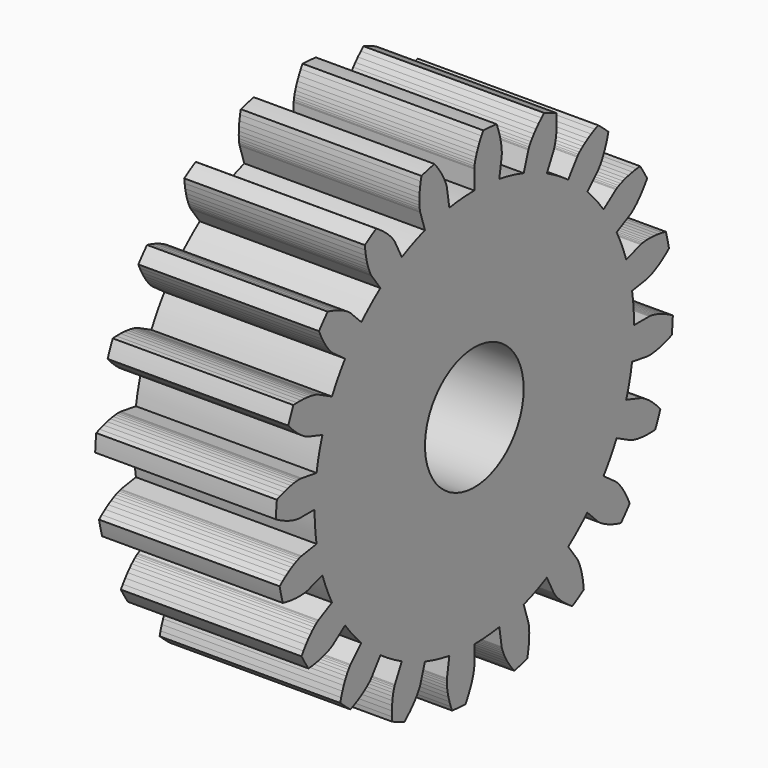
from build123d import *

# Parameters (mm, degrees)
F2_DEPTH = 12.7
F3_R     = 4.3353381976
F4_DEPTH = 12.701


# Not quite as in the source:
# - a variable given as a bare number and used for a length is read in inches; the dataset says mm whatever the document's units were


with BuildPart() as f2:
    # F1 (on Right) → F2 (new body)
    with BuildSketch(Plane.YZ):
        with BuildLine():
            ThreePointArc((13.8654281935, -2.1960680843), (13.9949872217, -1.1014293813), (14.0382625, 0))
            ThreePointArc((14.0382625, 0), (13.9949872217, 1.1014293813), (13.8654281935, 2.1960680843))
            ThreePointArc((13.8654281935, 2.1960680843), (13.6503841896, 3.2771672972), (13.3511810281, 4.338061684))
            ThreePointArc((13.3511810281, 4.338061684), (12.9696633958, 5.3722104779), (12.5081834758, 6.3732378078))
            ThreePointArc((12.5081834758, 6.3732378078), (11.9695864452, 7.3349720074), (11.357192934, 8.2514836653))
            ThreePointArc((11.357192934, 8.2514836653), (10.6747785517, 9.1171221826), (9.9265506098, 9.9265506098))
            ThreePointArc((9.9265506098, 9.9265506098), (9.1171221826, 10.6747785517), (8.2514836653, 11.357192934))
            ThreePointArc((8.2514836653, 11.357192934), (7.3349720074, 11.9695864452), (6.3732378078, 12.5081834758))
            ThreePointArc((6.3732378078, 12.5081834758), (5.3722104779, 12.9696633958), (4.338061684, 13.3511810281))
            ThreePointArc((4.338061684, 13.3511810281), (3.2771672972, 13.6503841896), (2.1960680843, 13.8654281935))
            ThreePointArc((2.1960680843, 13.8654281935), (1.1014293813, 13.9949872217), (0, 14.0382625))
            ThreePointArc((0, 14.0382625), (-1.1014293813, 13.9949872217), (-2.1960680843, 13.8654281935))
            ThreePointArc((-2.1960680843, 13.8654281935), (-3.2771672972, 13.6503841896), (-4.338061684, 13.3511810281))
            ThreePointArc((-4.338061684, 13.3511810281), (-5.3722104779, 12.9696633958), (-6.3732378078, 12.5081834758))
            ThreePointArc((-6.3732378078, 12.5081834758), (-7.3349720074, 11.9695864452), (-8.2514836653, 11.357192934))
            ThreePointArc((-8.2514836653, 11.357192934), (-9.1171221826, 10.6747785517), (-9.9265506098, 9.9265506098))
            ThreePointArc((-9.9265506098, 9.9265506098), (-10.6747785517, 9.1171221826), (-11.357192934, 8.2514836653))
            ThreePointArc((-11.357192934, 8.2514836653), (-11.9695864452, 7.3349720074), (-12.5081834758, 6.3732378078))
            ThreePointArc((-12.5081834758, 6.3732378078), (-12.9696633958, 5.3722104779), (-13.3511810281, 4.338061684))
            ThreePointArc((-13.3511810281, 4.338061684), (-13.6503841896, 3.2771672972), (-13.8654281935, 2.1960680843))
            ThreePointArc((-13.8654281935, 2.1960680843), (-13.9949872217, 1.1014293813), (-14.0382625, 0))
            ThreePointArc((-14.0382625, 0), (-13.9949872217, -1.1014293813), (-13.8654281935, -2.1960680843))
            ThreePointArc((-13.8654281935, -2.1960680843), (-13.6503841896, -3.2771672972), (-13.3511810281, -4.338061684))
            ThreePointArc((-13.3511810281, -4.338061684), (-12.9696633958, -5.3722104779), (-12.5081834758, -6.3732378078))
            ThreePointArc((-12.5081834758, -6.3732378078), (-11.9695864452, -7.3349720074), (-11.357192934, -8.2514836653))
            ThreePointArc((-11.357192934, -8.2514836653), (-10.6747785517, -9.1171221826), (-9.9265506098, -9.9265506098))
            ThreePointArc((-9.9265506098, -9.9265506098), (-9.1171221826, -10.6747785517), (-8.2514836653, -11.357192934))
            ThreePointArc((-8.2514836653, -11.357192934), (-7.3349720074, -11.9695864452), (-6.3732378078, -12.5081834758))
            ThreePointArc((-6.3732378078, -12.5081834758), (-5.3722104779, -12.9696633958), (-4.338061684, -13.3511810281))
            ThreePointArc((-4.338061684, -13.3511810281), (-3.2771672972, -13.6503841896), (-2.1960680843, -13.8654281935))
            ThreePointArc((-2.1960680843, -13.8654281935), (-1.1014293813, -13.9949872217), (0, -14.0382625))
            ThreePointArc((0, -14.0382625), (1.1014293813, -13.9949872217), (2.1960680843, -13.8654281935))
            ThreePointArc((2.1960680843, -13.8654281935), (3.2771672972, -13.6503841896), (4.338061684, -13.3511810281))
            ThreePointArc((4.338061684, -13.3511810281), (5.3722104779, -12.9696633958), (6.3732378078, -12.5081834758))
            ThreePointArc((6.3732378078, -12.5081834758), (7.3349720074, -11.9695864452), (8.2514836653, -11.357192934))
            ThreePointArc((8.2514836653, -11.357192934), (9.1171221826, -10.6747785517), (9.9265506098, -9.9265506098))
            ThreePointArc((9.9265506098, -9.9265506098), (10.6747785517, -9.1171221826), (11.357192934, -8.2514836653))
            ThreePointArc((11.357192934, -8.2514836653), (11.9695864452, -7.3349720074), (12.5081834758, -6.3732378078))
            ThreePointArc((12.5081834758, -6.3732378078), (12.9696633958, -5.3722104779), (13.3511810281, -4.338061684))
            ThreePointArc((13.3511810281, -4.338061684), (13.6503841896, -3.2771672972), (13.8654281935, -2.1960680843))
        make_face()
        with BuildLine():
            Line((-14.6171145636, -4.7493884238), (-13.3511810281, -4.338061684))
            ThreePointArc((-13.3511810281, -4.338061684), (-13.6503841896, -3.2771672972), (-13.8654281935, -2.1960680843))
            Line((-13.8654281935, -2.1960680843), (-15.180121665, -2.404295074))
            Line((-15.180121665, -2.404295074), (-15.1989848071, -2.4079309004))
            Line((-15.1989848071, -2.4079309004), (-15.2550320002, -2.4213414721))
            Line((-15.2550320002, -2.4213414721), (-15.3472398712, -2.4482306459))
            Line((-15.3472398712, -2.4482306459), (-15.474308977, -2.4922197725))
            Line((-15.474308977, -2.4922197725), (-15.6346697243, -2.5568294258))
            Line((-15.6346697243, -2.5568294258), (-15.8264894224, -2.6454615286))
            Line((-15.8264894224, -2.6454615286), (-16.0476804424, -2.7613819428))
            Line((-16.0476804424, -2.7613819428), (-16.2959094551, -2.9077035901))
            Line((-16.2959094551, -2.9077035901), (-16.5686077133, -3.0873701663))
            Line((-16.5686077133, -3.0873701663), (-16.8629823421, -3.3031405114))
            Line((-16.8629823421, -3.3031405114), (-17.1077308908, -3.5020636798))
            ThreePointArc((-17.1077308908, -3.5020636798), (-16.9800097349, -4.0765396663), (-16.8330034779, -4.6463857097))
            Line((-16.8330034779, -4.6463857097), (-16.5246216956, -4.7125140346))
            Line((-16.5246216956, -4.7125140346), (-16.1643742939, -4.771123535))
            Line((-16.1643742939, -4.771123535), (-15.8398314481, -4.807405208))
            Line((-15.8398314481, -4.807405208), (-15.5522291405, -4.8250851369))
            Line((-15.5522291405, -4.8250851369), (-15.3025197318, -4.8279523605))
            Line((-15.3025197318, -4.8279523605), (-15.0913689967, -4.8198398218))
            Line((-15.0913689967, -4.8198398218), (-14.9191543558, -4.8046051886))
            Line((-14.9191543558, -4.8046051886), (-14.7859643079, -4.7861116205))
            Line((-14.7859643079, -4.7861116205), (-14.6915990638, -4.7682085524))
            Line((-14.6915990638, -4.7682085524), (-14.635572377, -4.754712566))
            Line((-14.635572377, -4.754712566), (-14.6171145636, -4.7493884238))
        make_face()
        with BuildLine():
            Line((-12.4340603193, -9.0338736178), (-11.357192934, -8.2514836653))
            ThreePointArc((-11.357192934, -8.2514836653), (-11.9695864452, -7.3349720074), (-12.5081834758, -6.3732378078))
            Line((-12.5081834758, -6.3732378078), (-13.6941855903, -6.9775360683))
            Line((-13.6941855903, -6.9775360683), (-13.7110019723, -6.9868229763))
            Line((-13.7110019723, -6.9868229763), (-13.760161926, -7.016896723))
            Line((-13.760161926, -7.016896723), (-13.8395476109, -7.0709636461))
            Line((-13.8395476109, -7.0709636461), (-13.9468041243, -7.1520663048))
            Line((-13.9468041243, -7.1520663048), (-14.0793507771, -7.2630679327))
            Line((-14.0793507771, -7.2630679327), (-14.234393325, -7.4066376182))
            Line((-14.234393325, -7.4066376182), (-14.4089371079, -7.5852362677))
            Line((-14.4089371079, -7.5852362677), (-14.5998010523, -7.8011034073))
            Line((-14.5998010523, -7.8011034073), (-14.8036324824, -8.0562448714))
            Line((-14.8036324824, -8.0562448714), (-15.0169226878, -8.3524214272))
            Line((-15.0169226878, -8.3524214272), (-15.1882217503, -8.6172400636))
            ThreePointArc((-15.1882217503, -8.6172400636), (-14.88922887, -9.1241311864), (-14.5733254998, -9.6206595475))
            Line((-14.5733254998, -9.6206595475), (-14.25960222, -9.5882561103))
            Line((-14.25960222, -9.5882561103), (-13.8988752495, -9.5326744883))
            Line((-13.8988752495, -9.5326744883), (-13.5790050076, -9.466891155))
            Line((-13.5790050076, -9.466891155), (-13.3000155603, -9.3948317659))
            Line((-13.3000155603, -9.3948317659), (-13.0616417792, -9.3203942067))
            Line((-13.0616417792, -9.3203942067), (-12.863332409, -9.2474295583))
            Line((-12.863332409, -9.2474295583), (-12.7042543131, -9.1797233104))
            Line((-12.7042543131, -9.1797233104), (-12.583297877, -9.1209768938))
            Line((-12.583297877, -9.1209768938), (-12.4990835491, -9.0747896001))
            Line((-12.4990835491, -9.0747896001), (-12.4499694926, -9.0446409559))
            Line((-12.4499694926, -9.0446409559), (-12.4340603193, -9.0338736178))
        make_face()
        with BuildLine():
            Line((-9.0338736178, -12.4340603193), (-8.2514836653, -11.357192934))
            ThreePointArc((-8.2514836653, -11.357192934), (-9.1171221826, -10.6747785517), (-9.9265506098, -9.9265506098))
            Line((-9.9265506098, -9.9265506098), (-10.867767217, -10.867767217))
            Line((-10.867767217, -10.867767217), (-10.8808907344, -10.8817961392))
            Line((-10.8808907344, -10.8817961392), (-10.9183513298, -10.9255892331))
            Line((-10.9183513298, -10.9255892331), (-10.9771440047, -11.0015414583))
            Line((-10.9771440047, -11.0015414583), (-11.0540889108, -11.1118187557))
            Line((-11.0540889108, -11.1118187557), (-11.1458468793, -11.2583467456))
            Line((-11.1458468793, -11.2583467456), (-11.248935632, -11.4428004126))
            Line((-11.248935632, -11.4428004126), (-11.3597466163, -11.6665948172))
            Line((-11.3597466163, -11.6665948172), (-11.4745623996, -11.9308768694))
            Line((-11.4745623996, -11.9308768694), (-11.5895745611, -12.2365181973))
            Line((-11.5895745611, -12.2365181973), (-11.7009020117, -12.5841091389))
            Line((-11.7009020117, -12.5841091389), (-11.7819836423, -12.8889009502))
            ThreePointArc((-11.7819836423, -12.8889009502), (-11.340986544, -13.2785891743), (-10.8871088834, -13.6531961976))
            Line((-10.8871088834, -13.6531961976), (-10.5987535266, -13.5254328726))
            Line((-10.5987535266, -13.5254328726), (-10.2728574565, -13.3611008446))
            Line((-10.2728574565, -13.3611008446), (-9.9889709465, -13.1996918361))
            Line((-9.9889709465, -13.1996918361), (-9.7459037905, -13.0449468041))
            Line((-9.7459037905, -13.0449468041), (-9.5421993235, -12.900490929))
            Line((-9.5421993235, -12.900490929), (-9.3761432211, -12.7698164591))
            Line((-9.3761432211, -12.7698164591), (-9.2457733426, -12.6562661558))
            Line((-9.2457733426, -12.6562661558), (-9.1488905769, -12.5630173991))
            Line((-9.1488905769, -12.5630173991), (-9.0830706503, -12.4930670139))
            Line((-9.0830706503, -12.4930670139), (-9.0456768502, -12.4492168713))
            Line((-9.0456768502, -12.4492168713), (-9.0338736178, -12.4340603193))
        make_face()
        with BuildLine():
            Line((-4.7493884238, -14.6171145636), (-4.338061684, -13.3511810281))
            ThreePointArc((-4.338061684, -13.3511810281), (-5.3722104779, -12.9696633958), (-6.3732378078, -12.5081834758))
            Line((-6.3732378078, -12.5081834758), (-6.9775360683, -13.6941855903))
            Line((-6.9775360683, -13.6941855903), (-6.9856820997, -13.711583278))
            Line((-6.9856820997, -13.711583278), (-7.0077764328, -13.764808946))
            Line((-7.0077764328, -13.764808946), (-7.040221061, -13.8552117404))
            Line((-7.040221061, -13.8552117404), (-7.0793224564, -13.9838689663))
            Line((-7.0793224564, -13.9838689663), (-7.1213098312, -14.1515801375))
            Line((-7.1213098312, -14.1515801375), (-7.1623537435, -14.358862176))
            Line((-7.1623537435, -14.358862176), (-7.1985849778, -14.6059457801))
            Line((-7.1985849778, -14.6059457801), (-7.2261136314, -14.8927729763))
            Line((-7.2261136314, -14.8927729763), (-7.2410483324, -15.2189958653))
            Line((-7.2410483324, -15.2189958653), (-7.2395155218, -15.5839765695))
            Line((-7.2395155218, -15.5839765695), (-7.2224428854, -15.8989064095))
            ThreePointArc((-7.2224428854, -15.8989064095), (-6.6826094377, -16.1332463365), (-6.1351861945, -16.3492628766))
            Line((-6.1351861945, -16.3492628766), (-5.9004249921, -16.1386460281))
            Line((-5.9004249921, -16.1386460281), (-5.6412608004, -15.881649558))
            Line((-5.6412608004, -15.881649558), (-5.4211468118, -15.6404147126))
            Line((-5.4211468118, -15.6404147126), (-5.237795054, -15.4181315596))
            Line((-5.237795054, -15.4181315596), (-5.0886999135, -15.2177977161))
            Line((-5.0886999135, -15.2177977161), (-4.9711518072, -15.0422047523))
            Line((-4.9711518072, -15.0422047523), (-4.8822516582, -14.8939254884))
            Line((-4.8822516582, -14.8939254884), (-4.8189261231, -14.7753022297))
            Line((-4.8189261231, -14.7753022297), (-4.7779435107, -14.6884359841))
            Line((-4.7779435107, -14.6884359841), (-4.7559303328, -14.6351767006))
            Line((-4.7559303328, -14.6351767006), (-4.7493884238, -14.6171145636))
        make_face()
        with BuildLine():
            Line((0, -15.369343791), (0, -14.0382625))
            ThreePointArc((0, -14.0382625), (-1.1014293813, -13.9949872217), (-2.1960680843, -13.8654281935))
            Line((-2.1960680843, -13.8654281935), (-2.404295074, -15.180121665))
            Line((-2.404295074, -15.180121665), (-2.406666229, -15.1991851114))
            Line((-2.406666229, -15.1991851114), (-2.4112315526, -15.2566332542))
            Line((-2.4112315526, -15.2566332542), (-2.4141522278, -15.3526373623))
            Line((-2.4141522278, -15.3526373623), (-2.4115825954, -15.4870806511))
            Line((-2.4115825954, -15.4870806511), (-2.3996893598, -15.6595582657))
            Line((-2.3996893598, -15.6595582657), (-2.3746707675, -15.8693784656))
            Line((-2.3746707675, -15.8693784656), (-2.3327756863, -16.1155650045))
            Line((-2.3327756863, -16.1155650045), (-2.2703225136, -16.3968607002))
            Line((-2.2703225136, -16.3968607002), (-2.1837178417, -16.711732181))
            Line((-2.1837178417, -16.711732181), (-2.0694748119, -17.0583757934))
            Line((-2.0694748119, -17.0583757934), (-1.9559190973, -17.3526161352))
            ThreePointArc((-1.9559190973, -17.3526161352), (-1.3700919591, -17.4086689403), (-0.7827087346, -17.4449497932))
            Line((-0.7827087346, -17.4449497932), (-0.6245217488, -17.1720960658))
            Line((-0.6245217488, -17.1720960658), (-0.4574582322, -16.8475917587))
            Line((-0.4574582322, -16.8475917587), (-0.3226630559, -16.5501448238))
            Line((-0.3226630559, -16.5501448238), (-0.2169744437, -16.2820821735))
            Line((-0.2169744437, -16.2820821735), (-0.137083101, -16.0454804341))
            Line((-0.137083101, -16.0454804341), (-0.0795494184, -15.8421572392))
            Line((-0.0795494184, -15.8421572392), (-0.0408211648, -15.6736636222))
            Line((-0.0408211648, -15.6736636222), (-0.0172516049, -15.5412775325))
            Line((-0.0172516049, -15.5412775325), (-0.0051179705, -15.4459984999))
            Line((-0.0051179705, -15.4459984999), (-0.0006402179, -15.3885434651))
            Line((-0.0006402179, -15.3885434651), (0, -15.369343791))
        make_face()
        with BuildLine():
            Line((4.7493884238, -14.6171145636), (4.338061684, -13.3511810281))
            ThreePointArc((4.338061684, -13.3511810281), (3.2771672972, -13.6503841896), (2.1960680843, -13.8654281935))
            Line((2.1960680843, -13.8654281935), (2.404295074, -15.180121665))
            Line((2.404295074, -15.180121665), (2.4079309004, -15.1989848071))
            Line((2.4079309004, -15.1989848071), (2.4213414721, -15.2550320002))
            Line((2.4213414721, -15.2550320002), (2.4482306459, -15.3472398712))
            Line((2.4482306459, -15.3472398712), (2.4922197725, -15.474308977))
            Line((2.4922197725, -15.474308977), (2.5568294258, -15.6346697243))
            Line((2.5568294258, -15.6346697243), (2.6454615286, -15.8264894224))
            Line((2.6454615286, -15.8264894224), (2.7613819428, -16.0476804424))
            Line((2.7613819428, -16.0476804424), (2.9077035901, -16.2959094551))
            Line((2.9077035901, -16.2959094551), (3.0873701663, -16.5686077133))
            Line((3.0873701663, -16.5686077133), (3.3031405114, -16.8629823421))
            Line((3.3031405114, -16.8629823421), (3.5020636798, -17.1077308908))
            ThreePointArc((3.5020636798, -17.1077308908), (4.0765396663, -16.9800097349), (4.6463857097, -16.8330034779))
            Line((4.6463857097, -16.8330034779), (4.7125140346, -16.5246216956))
            Line((4.7125140346, -16.5246216956), (4.771123535, -16.1643742939))
            Line((4.771123535, -16.1643742939), (4.807405208, -15.8398314481))
            Line((4.807405208, -15.8398314481), (4.8250851369, -15.5522291405))
            Line((4.8250851369, -15.5522291405), (4.8279523605, -15.3025197318))
            Line((4.8279523605, -15.3025197318), (4.8198398218, -15.0913689967))
            Line((4.8198398218, -15.0913689967), (4.8046051886, -14.9191543558))
            Line((4.8046051886, -14.9191543558), (4.7861116205, -14.7859643079))
            Line((4.7861116205, -14.7859643079), (4.7682085524, -14.6915990638))
            Line((4.7682085524, -14.6915990638), (4.754712566, -14.635572377))
            Line((4.754712566, -14.635572377), (4.7493884238, -14.6171145636))
        make_face()
        with BuildLine():
            Line((9.0338736178, -12.4340603193), (8.2514836653, -11.357192934))
            ThreePointArc((8.2514836653, -11.357192934), (7.3349720074, -11.9695864452), (6.3732378078, -12.5081834758))
            Line((6.3732378078, -12.5081834758), (6.9775360683, -13.6941855903))
            Line((6.9775360683, -13.6941855903), (6.9868229763, -13.7110019723))
            Line((6.9868229763, -13.7110019723), (7.016896723, -13.760161926))
            Line((7.016896723, -13.760161926), (7.0709636461, -13.8395476109))
            Line((7.0709636461, -13.8395476109), (7.1520663048, -13.9468041243))
            Line((7.1520663048, -13.9468041243), (7.2630679327, -14.0793507771))
            Line((7.2630679327, -14.0793507771), (7.4066376182, -14.234393325))
            Line((7.4066376182, -14.234393325), (7.5852362677, -14.4089371079))
            Line((7.5852362677, -14.4089371079), (7.8011034073, -14.5998010523))
            Line((7.8011034073, -14.5998010523), (8.0562448714, -14.8036324824))
            Line((8.0562448714, -14.8036324824), (8.3524214272, -15.0169226878))
            Line((8.3524214272, -15.0169226878), (8.6172400636, -15.1882217503))
            ThreePointArc((8.6172400636, -15.1882217503), (9.1241311864, -14.88922887), (9.6206595475, -14.5733254998))
            Line((9.6206595475, -14.5733254998), (9.5882561103, -14.25960222))
            Line((9.5882561103, -14.25960222), (9.5326744883, -13.8988752495))
            Line((9.5326744883, -13.8988752495), (9.466891155, -13.5790050076))
            Line((9.466891155, -13.5790050076), (9.3948317659, -13.3000155603))
            Line((9.3948317659, -13.3000155603), (9.3203942067, -13.0616417792))
            Line((9.3203942067, -13.0616417792), (9.2474295583, -12.863332409))
            Line((9.2474295583, -12.863332409), (9.1797233104, -12.7042543131))
            Line((9.1797233104, -12.7042543131), (9.1209768938, -12.583297877))
            Line((9.1209768938, -12.583297877), (9.0747896001, -12.4990835491))
            Line((9.0747896001, -12.4990835491), (9.0446409559, -12.4499694926))
            Line((9.0446409559, -12.4499694926), (9.0338736178, -12.4340603193))
        make_face()
        with BuildLine():
            Line((12.4340603193, -9.0338736178), (11.357192934, -8.2514836653))
            ThreePointArc((11.357192934, -8.2514836653), (10.6747785517, -9.1171221826), (9.9265506098, -9.9265506098))
            Line((9.9265506098, -9.9265506098), (10.867767217, -10.867767217))
            Line((10.867767217, -10.867767217), (10.8817961392, -10.8808907344))
            Line((10.8817961392, -10.8808907344), (10.9255892331, -10.9183513298))
            Line((10.9255892331, -10.9183513298), (11.0015414583, -10.9771440047))
            Line((11.0015414583, -10.9771440047), (11.1118187557, -11.0540889108))
            Line((11.1118187557, -11.0540889108), (11.2583467456, -11.1458468793))
            Line((11.2583467456, -11.1458468793), (11.4428004126, -11.248935632))
            Line((11.4428004126, -11.248935632), (11.6665948172, -11.3597466163))
            Line((11.6665948172, -11.3597466163), (11.9308768694, -11.4745623996))
            Line((11.9308768694, -11.4745623996), (12.2365181973, -11.5895745611))
            Line((12.2365181973, -11.5895745611), (12.5841091389, -11.7009020117))
            Line((12.5841091389, -11.7009020117), (12.8889009502, -11.7819836423))
            ThreePointArc((12.8889009502, -11.7819836423), (13.2785891743, -11.340986544), (13.6531961976, -10.8871088834))
            Line((13.6531961976, -10.8871088834), (13.5254328726, -10.5987535266))
            Line((13.5254328726, -10.5987535266), (13.3611008446, -10.2728574565))
            Line((13.3611008446, -10.2728574565), (13.1996918361, -9.9889709465))
            Line((13.1996918361, -9.9889709465), (13.0449468041, -9.7459037905))
            Line((13.0449468041, -9.7459037905), (12.900490929, -9.5421993235))
            Line((12.900490929, -9.5421993235), (12.7698164591, -9.3761432211))
            Line((12.7698164591, -9.3761432211), (12.6562661558, -9.2457733426))
            Line((12.6562661558, -9.2457733426), (12.5630173991, -9.1488905769))
            Line((12.5630173991, -9.1488905769), (12.4930670139, -9.0830706503))
            Line((12.4930670139, -9.0830706503), (12.4492168713, -9.0456768502))
            Line((12.4492168713, -9.0456768502), (12.4340603193, -9.0338736178))
        make_face()
        with BuildLine():
            Line((14.6171145636, -4.7493884238), (13.3511810281, -4.338061684))
            ThreePointArc((13.3511810281, -4.338061684), (12.9696633958, -5.3722104779), (12.5081834758, -6.3732378078))
            Line((12.5081834758, -6.3732378078), (13.6941855903, -6.9775360683))
            Line((13.6941855903, -6.9775360683), (13.711583278, -6.9856820997))
            Line((13.711583278, -6.9856820997), (13.764808946, -7.0077764328))
            Line((13.764808946, -7.0077764328), (13.8552117404, -7.040221061))
            Line((13.8552117404, -7.040221061), (13.9838689663, -7.0793224564))
            Line((13.9838689663, -7.0793224564), (14.1515801375, -7.1213098312))
            Line((14.1515801375, -7.1213098312), (14.358862176, -7.1623537435))
            Line((14.358862176, -7.1623537435), (14.6059457801, -7.1985849778))
            Line((14.6059457801, -7.1985849778), (14.8927729763, -7.2261136314))
            Line((14.8927729763, -7.2261136314), (15.2189958653, -7.2410483324))
            Line((15.2189958653, -7.2410483324), (15.5839765695, -7.2395155218))
            Line((15.5839765695, -7.2395155218), (15.8989064095, -7.2224428854))
            ThreePointArc((15.8989064095, -7.2224428854), (16.1332463365, -6.6826094377), (16.3492628766, -6.1351861945))
            Line((16.3492628766, -6.1351861945), (16.1386460281, -5.9004249921))
            Line((16.1386460281, -5.9004249921), (15.881649558, -5.6412608004))
            Line((15.881649558, -5.6412608004), (15.6404147126, -5.4211468118))
            Line((15.6404147126, -5.4211468118), (15.4181315596, -5.237795054))
            Line((15.4181315596, -5.237795054), (15.2177977161, -5.0886999135))
            Line((15.2177977161, -5.0886999135), (15.0422047523, -4.9711518072))
            Line((15.0422047523, -4.9711518072), (14.8939254884, -4.8822516582))
            Line((14.8939254884, -4.8822516582), (14.7753022297, -4.8189261231))
            Line((14.7753022297, -4.8189261231), (14.6884359841, -4.7779435107))
            Line((14.6884359841, -4.7779435107), (14.6351767006, -4.7559303328))
            Line((14.6351767006, -4.7559303328), (14.6171145636, -4.7493884238))
        make_face()
        with BuildLine():
            Line((15.369343791, 0), (14.0382625, 0))
            ThreePointArc((14.0382625, 0), (13.9949872217, -1.1014293813), (13.8654281935, -2.1960680843))
            Line((13.8654281935, -2.1960680843), (15.180121665, -2.404295074))
            Line((15.180121665, -2.404295074), (15.1991851114, -2.406666229))
            Line((15.1991851114, -2.406666229), (15.2566332542, -2.4112315526))
            Line((15.2566332542, -2.4112315526), (15.3526373623, -2.4141522278))
            Line((15.3526373623, -2.4141522278), (15.4870806511, -2.4115825954))
            Line((15.4870806511, -2.4115825954), (15.6595582657, -2.3996893598))
            Line((15.6595582657, -2.3996893598), (15.8693784656, -2.3746707675))
            Line((15.8693784656, -2.3746707675), (16.1155650045, -2.3327756863))
            Line((16.1155650045, -2.3327756863), (16.3968607002, -2.2703225136))
            Line((16.3968607002, -2.2703225136), (16.711732181, -2.1837178417))
            Line((16.711732181, -2.1837178417), (17.0583757934, -2.0694748119))
            Line((17.0583757934, -2.0694748119), (17.3526161352, -1.9559190973))
            ThreePointArc((17.3526161352, -1.9559190973), (17.4086689403, -1.3700919591), (17.4449497932, -0.7827087346))
            Line((17.4449497932, -0.7827087346), (17.1720960658, -0.6245217488))
            Line((17.1720960658, -0.6245217488), (16.8475917587, -0.4574582322))
            Line((16.8475917587, -0.4574582322), (16.5501448238, -0.3226630559))
            Line((16.5501448238, -0.3226630559), (16.2820821735, -0.2169744437))
            Line((16.2820821735, -0.2169744437), (16.0454804341, -0.137083101))
            Line((16.0454804341, -0.137083101), (15.8421572392, -0.0795494184))
            Line((15.8421572392, -0.0795494184), (15.6736636222, -0.0408211648))
            Line((15.6736636222, -0.0408211648), (15.5412775325, -0.0172516049))
            Line((15.5412775325, -0.0172516049), (15.4459984999, -0.0051179705))
            Line((15.4459984999, -0.0051179705), (15.3885434651, -0.0006402179))
            Line((15.3885434651, -0.0006402179), (15.369343791, 0))
        make_face()
        with BuildLine():
            ThreePointArc((13.3511810281, 4.338061684), (13.6503841896, 3.2771672972), (13.8654281935, 2.1960680843))
            Line((13.8654281935, 2.1960680843), (15.180121665, 2.404295074))
            Line((15.180121665, 2.404295074), (15.1989848071, 2.4079309004))
            Line((15.1989848071, 2.4079309004), (15.2550320002, 2.4213414721))
            Line((15.2550320002, 2.4213414721), (15.3472398712, 2.4482306459))
            Line((15.3472398712, 2.4482306459), (15.474308977, 2.4922197725))
            Line((15.474308977, 2.4922197725), (15.6346697243, 2.5568294258))
            Line((15.6346697243, 2.5568294258), (15.8264894224, 2.6454615286))
            Line((15.8264894224, 2.6454615286), (16.0476804424, 2.7613819428))
            Line((16.0476804424, 2.7613819428), (16.2959094551, 2.9077035901))
            Line((16.2959094551, 2.9077035901), (16.5686077133, 3.0873701663))
            Line((16.5686077133, 3.0873701663), (16.8629823421, 3.3031405114))
            Line((16.8629823421, 3.3031405114), (17.1077308908, 3.5020636798))
            ThreePointArc((17.1077308908, 3.5020636798), (16.9800097349, 4.0765396663), (16.8330034779, 4.6463857097))
            Line((16.8330034779, 4.6463857097), (16.5246216956, 4.7125140346))
            Line((16.5246216956, 4.7125140346), (16.1643742939, 4.771123535))
            Line((16.1643742939, 4.771123535), (15.8398314481, 4.807405208))
            Line((15.8398314481, 4.807405208), (15.5522291405, 4.8250851369))
            Line((15.5522291405, 4.8250851369), (15.3025197318, 4.8279523605))
            Line((15.3025197318, 4.8279523605), (15.0913689967, 4.8198398218))
            Line((15.0913689967, 4.8198398218), (14.9191543558, 4.8046051886))
            Line((14.9191543558, 4.8046051886), (14.7859643079, 4.7861116205))
            Line((14.7859643079, 4.7861116205), (14.6915990638, 4.7682085524))
            Line((14.6915990638, 4.7682085524), (14.635572377, 4.754712566))
            Line((14.635572377, 4.754712566), (14.6171145636, 4.7493884238))
            Line((14.6171145636, 4.7493884238), (13.3511810281, 4.338061684))
        make_face()
        with BuildLine():
            ThreePointArc((11.357192934, 8.2514836653), (11.9695864452, 7.3349720074), (12.5081834758, 6.3732378078))
            Line((12.5081834758, 6.3732378078), (13.6941855903, 6.9775360683))
            Line((13.6941855903, 6.9775360683), (13.7110019723, 6.9868229763))
            Line((13.7110019723, 6.9868229763), (13.760161926, 7.016896723))
            Line((13.760161926, 7.016896723), (13.8395476109, 7.0709636461))
            Line((13.8395476109, 7.0709636461), (13.9468041243, 7.1520663048))
            Line((13.9468041243, 7.1520663048), (14.0793507771, 7.2630679327))
            Line((14.0793507771, 7.2630679327), (14.234393325, 7.4066376182))
            Line((14.234393325, 7.4066376182), (14.4089371079, 7.5852362677))
            Line((14.4089371079, 7.5852362677), (14.5998010523, 7.8011034073))
            Line((14.5998010523, 7.8011034073), (14.8036324824, 8.0562448714))
            Line((14.8036324824, 8.0562448714), (15.0169226878, 8.3524214272))
            Line((15.0169226878, 8.3524214272), (15.1882217503, 8.6172400636))
            ThreePointArc((15.1882217503, 8.6172400636), (14.88922887, 9.1241311864), (14.5733254998, 9.6206595475))
            Line((14.5733254998, 9.6206595475), (14.25960222, 9.5882561103))
            Line((14.25960222, 9.5882561103), (13.8988752495, 9.5326744883))
            Line((13.8988752495, 9.5326744883), (13.5790050076, 9.466891155))
            Line((13.5790050076, 9.466891155), (13.3000155603, 9.3948317659))
            Line((13.3000155603, 9.3948317659), (13.0616417792, 9.3203942067))
            Line((13.0616417792, 9.3203942067), (12.863332409, 9.2474295583))
            Line((12.863332409, 9.2474295583), (12.7042543131, 9.1797233104))
            Line((12.7042543131, 9.1797233104), (12.583297877, 9.1209768938))
            Line((12.583297877, 9.1209768938), (12.4990835491, 9.0747896001))
            Line((12.4990835491, 9.0747896001), (12.4499694926, 9.0446409559))
            Line((12.4499694926, 9.0446409559), (12.4340603193, 9.0338736178))
            Line((12.4340603193, 9.0338736178), (11.357192934, 8.2514836653))
        make_face()
        with BuildLine():
            ThreePointArc((8.2514836653, 11.357192934), (9.1171221826, 10.6747785517), (9.9265506098, 9.9265506098))
            Line((9.9265506098, 9.9265506098), (10.867767217, 10.867767217))
            Line((10.867767217, 10.867767217), (10.8808907344, 10.8817961392))
            Line((10.8808907344, 10.8817961392), (10.9183513298, 10.9255892331))
            Line((10.9183513298, 10.9255892331), (10.9771440047, 11.0015414583))
            Line((10.9771440047, 11.0015414583), (11.0540889108, 11.1118187557))
            Line((11.0540889108, 11.1118187557), (11.1458468793, 11.2583467456))
            Line((11.1458468793, 11.2583467456), (11.248935632, 11.4428004126))
            Line((11.248935632, 11.4428004126), (11.3597466163, 11.6665948172))
            Line((11.3597466163, 11.6665948172), (11.4745623996, 11.9308768694))
            Line((11.4745623996, 11.9308768694), (11.5895745611, 12.2365181973))
            Line((11.5895745611, 12.2365181973), (11.7009020117, 12.5841091389))
            Line((11.7009020117, 12.5841091389), (11.7819836423, 12.8889009502))
            ThreePointArc((11.7819836423, 12.8889009502), (11.340986544, 13.2785891743), (10.8871088834, 13.6531961976))
            Line((10.8871088834, 13.6531961976), (10.5987535266, 13.5254328726))
            Line((10.5987535266, 13.5254328726), (10.2728574565, 13.3611008446))
            Line((10.2728574565, 13.3611008446), (9.9889709465, 13.1996918361))
            Line((9.9889709465, 13.1996918361), (9.7459037905, 13.0449468041))
            Line((9.7459037905, 13.0449468041), (9.5421993235, 12.900490929))
            Line((9.5421993235, 12.900490929), (9.3761432211, 12.7698164591))
            Line((9.3761432211, 12.7698164591), (9.2457733426, 12.6562661558))
            Line((9.2457733426, 12.6562661558), (9.1488905769, 12.5630173991))
            Line((9.1488905769, 12.5630173991), (9.0830706503, 12.4930670139))
            Line((9.0830706503, 12.4930670139), (9.0456768502, 12.4492168713))
            Line((9.0456768502, 12.4492168713), (9.0338736178, 12.4340603193))
            Line((9.0338736178, 12.4340603193), (8.2514836653, 11.357192934))
        make_face()
        with BuildLine():
            ThreePointArc((4.338061684, 13.3511810281), (5.3722104779, 12.9696633958), (6.3732378078, 12.5081834758))
            Line((6.3732378078, 12.5081834758), (6.9775360683, 13.6941855903))
            Line((6.9775360683, 13.6941855903), (6.9856820997, 13.711583278))
            Line((6.9856820997, 13.711583278), (7.0077764328, 13.764808946))
            Line((7.0077764328, 13.764808946), (7.040221061, 13.8552117404))
            Line((7.040221061, 13.8552117404), (7.0793224564, 13.9838689663))
            Line((7.0793224564, 13.9838689663), (7.1213098312, 14.1515801375))
            Line((7.1213098312, 14.1515801375), (7.1623537435, 14.358862176))
            Line((7.1623537435, 14.358862176), (7.1985849778, 14.6059457801))
            Line((7.1985849778, 14.6059457801), (7.2261136314, 14.8927729763))
            Line((7.2261136314, 14.8927729763), (7.2410483324, 15.2189958653))
            Line((7.2410483324, 15.2189958653), (7.2395155218, 15.5839765695))
            Line((7.2395155218, 15.5839765695), (7.2224428854, 15.8989064095))
            ThreePointArc((7.2224428854, 15.8989064095), (6.6826094377, 16.1332463365), (6.1351861945, 16.3492628766))
            Line((6.1351861945, 16.3492628766), (5.9004249921, 16.1386460281))
            Line((5.9004249921, 16.1386460281), (5.6412608004, 15.881649558))
            Line((5.6412608004, 15.881649558), (5.4211468118, 15.6404147126))
            Line((5.4211468118, 15.6404147126), (5.237795054, 15.4181315596))
            Line((5.237795054, 15.4181315596), (5.0886999135, 15.2177977161))
            Line((5.0886999135, 15.2177977161), (4.9711518072, 15.0422047523))
            Line((4.9711518072, 15.0422047523), (4.8822516582, 14.8939254884))
            Line((4.8822516582, 14.8939254884), (4.8189261231, 14.7753022297))
            Line((4.8189261231, 14.7753022297), (4.7779435107, 14.6884359841))
            Line((4.7779435107, 14.6884359841), (4.7559303328, 14.6351767006))
            Line((4.7559303328, 14.6351767006), (4.7493884238, 14.6171145636))
            Line((4.7493884238, 14.6171145636), (4.338061684, 13.3511810281))
        make_face()
        with BuildLine():
            ThreePointArc((0, 14.0382625), (1.1014293813, 13.9949872217), (2.1960680843, 13.8654281935))
            Line((2.1960680843, 13.8654281935), (2.404295074, 15.180121665))
            Line((2.404295074, 15.180121665), (2.406666229, 15.1991851114))
            Line((2.406666229, 15.1991851114), (2.4112315526, 15.2566332542))
            Line((2.4112315526, 15.2566332542), (2.4141522278, 15.3526373623))
            Line((2.4141522278, 15.3526373623), (2.4115825954, 15.4870806511))
            Line((2.4115825954, 15.4870806511), (2.3996893598, 15.6595582657))
            Line((2.3996893598, 15.6595582657), (2.3746707675, 15.8693784656))
            Line((2.3746707675, 15.8693784656), (2.3327756863, 16.1155650045))
            Line((2.3327756863, 16.1155650045), (2.2703225136, 16.3968607002))
            Line((2.2703225136, 16.3968607002), (2.1837178417, 16.711732181))
            Line((2.1837178417, 16.711732181), (2.0694748119, 17.0583757934))
            Line((2.0694748119, 17.0583757934), (1.9559190973, 17.3526161352))
            ThreePointArc((1.9559190973, 17.3526161352), (1.3700919591, 17.4086689403), (0.7827087346, 17.4449497932))
            Line((0.7827087346, 17.4449497932), (0.6245217488, 17.1720960658))
            Line((0.6245217488, 17.1720960658), (0.4574582322, 16.8475917587))
            Line((0.4574582322, 16.8475917587), (0.3226630559, 16.5501448238))
            Line((0.3226630559, 16.5501448238), (0.2169744437, 16.2820821735))
            Line((0.2169744437, 16.2820821735), (0.137083101, 16.0454804341))
            Line((0.137083101, 16.0454804341), (0.0795494184, 15.8421572392))
            Line((0.0795494184, 15.8421572392), (0.0408211648, 15.6736636222))
            Line((0.0408211648, 15.6736636222), (0.0172516049, 15.5412775325))
            Line((0.0172516049, 15.5412775325), (0.0051179705, 15.4459984999))
            Line((0.0051179705, 15.4459984999), (0.0006402179, 15.3885434651))
            Line((0.0006402179, 15.3885434651), (0, 15.369343791))
            Line((0, 15.369343791), (0, 14.0382625))
        make_face()
        with BuildLine():
            ThreePointArc((-4.338061684, 13.3511810281), (-3.2771672972, 13.6503841896), (-2.1960680843, 13.8654281935))
            Line((-2.1960680843, 13.8654281935), (-2.404295074, 15.180121665))
            Line((-2.404295074, 15.180121665), (-2.4079309004, 15.1989848071))
            Line((-2.4079309004, 15.1989848071), (-2.4213414721, 15.2550320002))
            Line((-2.4213414721, 15.2550320002), (-2.4482306459, 15.3472398712))
            Line((-2.4482306459, 15.3472398712), (-2.4922197725, 15.474308977))
            Line((-2.4922197725, 15.474308977), (-2.5568294258, 15.6346697243))
            Line((-2.5568294258, 15.6346697243), (-2.6454615286, 15.8264894224))
            Line((-2.6454615286, 15.8264894224), (-2.7613819428, 16.0476804424))
            Line((-2.7613819428, 16.0476804424), (-2.9077035901, 16.2959094551))
            Line((-2.9077035901, 16.2959094551), (-3.0873701663, 16.5686077133))
            Line((-3.0873701663, 16.5686077133), (-3.3031405114, 16.8629823421))
            Line((-3.3031405114, 16.8629823421), (-3.5020636798, 17.1077308908))
            ThreePointArc((-3.5020636798, 17.1077308908), (-4.0765396663, 16.9800097349), (-4.6463857097, 16.8330034779))
            Line((-4.6463857097, 16.8330034779), (-4.7125140346, 16.5246216956))
            Line((-4.7125140346, 16.5246216956), (-4.771123535, 16.1643742939))
            Line((-4.771123535, 16.1643742939), (-4.807405208, 15.8398314481))
            Line((-4.807405208, 15.8398314481), (-4.8250851369, 15.5522291405))
            Line((-4.8250851369, 15.5522291405), (-4.8279523605, 15.3025197318))
            Line((-4.8279523605, 15.3025197318), (-4.8198398218, 15.0913689967))
            Line((-4.8198398218, 15.0913689967), (-4.8046051886, 14.9191543558))
            Line((-4.8046051886, 14.9191543558), (-4.7861116205, 14.7859643079))
            Line((-4.7861116205, 14.7859643079), (-4.7682085524, 14.6915990638))
            Line((-4.7682085524, 14.6915990638), (-4.754712566, 14.635572377))
            Line((-4.754712566, 14.635572377), (-4.7493884238, 14.6171145636))
            Line((-4.7493884238, 14.6171145636), (-4.338061684, 13.3511810281))
        make_face()
        with BuildLine():
            ThreePointArc((-8.2514836653, 11.357192934), (-7.3349720074, 11.9695864452), (-6.3732378078, 12.5081834758))
            Line((-6.3732378078, 12.5081834758), (-6.9775360683, 13.6941855903))
            Line((-6.9775360683, 13.6941855903), (-6.9868229763, 13.7110019723))
            Line((-6.9868229763, 13.7110019723), (-7.016896723, 13.760161926))
            Line((-7.016896723, 13.760161926), (-7.0709636461, 13.8395476109))
            Line((-7.0709636461, 13.8395476109), (-7.1520663048, 13.9468041243))
            Line((-7.1520663048, 13.9468041243), (-7.2630679327, 14.0793507771))
            Line((-7.2630679327, 14.0793507771), (-7.4066376182, 14.234393325))
            Line((-7.4066376182, 14.234393325), (-7.5852362677, 14.4089371079))
            Line((-7.5852362677, 14.4089371079), (-7.8011034073, 14.5998010523))
            Line((-7.8011034073, 14.5998010523), (-8.0562448714, 14.8036324824))
            Line((-8.0562448714, 14.8036324824), (-8.3524214272, 15.0169226878))
            Line((-8.3524214272, 15.0169226878), (-8.6172400636, 15.1882217503))
            ThreePointArc((-8.6172400636, 15.1882217503), (-9.1241311864, 14.88922887), (-9.6206595475, 14.5733254998))
            Line((-9.6206595475, 14.5733254998), (-9.5882561103, 14.25960222))
            Line((-9.5882561103, 14.25960222), (-9.5326744883, 13.8988752495))
            Line((-9.5326744883, 13.8988752495), (-9.466891155, 13.5790050076))
            Line((-9.466891155, 13.5790050076), (-9.3948317659, 13.3000155603))
            Line((-9.3948317659, 13.3000155603), (-9.3203942067, 13.0616417792))
            Line((-9.3203942067, 13.0616417792), (-9.2474295583, 12.863332409))
            Line((-9.2474295583, 12.863332409), (-9.1797233104, 12.7042543131))
            Line((-9.1797233104, 12.7042543131), (-9.1209768938, 12.583297877))
            Line((-9.1209768938, 12.583297877), (-9.0747896001, 12.4990835491))
            Line((-9.0747896001, 12.4990835491), (-9.0446409559, 12.4499694926))
            Line((-9.0446409559, 12.4499694926), (-9.0338736178, 12.4340603193))
            Line((-9.0338736178, 12.4340603193), (-8.2514836653, 11.357192934))
        make_face()
        with BuildLine():
            ThreePointArc((-11.357192934, 8.2514836653), (-10.6747785517, 9.1171221826), (-9.9265506098, 9.9265506098))
            Line((-9.9265506098, 9.9265506098), (-10.867767217, 10.867767217))
            Line((-10.867767217, 10.867767217), (-10.8817961392, 10.8808907344))
            Line((-10.8817961392, 10.8808907344), (-10.9255892331, 10.9183513298))
            Line((-10.9255892331, 10.9183513298), (-11.0015414583, 10.9771440047))
            Line((-11.0015414583, 10.9771440047), (-11.1118187557, 11.0540889108))
            Line((-11.1118187557, 11.0540889108), (-11.2583467456, 11.1458468793))
            Line((-11.2583467456, 11.1458468793), (-11.4428004126, 11.248935632))
            Line((-11.4428004126, 11.248935632), (-11.6665948172, 11.3597466163))
            Line((-11.6665948172, 11.3597466163), (-11.9308768694, 11.4745623996))
            Line((-11.9308768694, 11.4745623996), (-12.2365181973, 11.5895745611))
            Line((-12.2365181973, 11.5895745611), (-12.5841091389, 11.7009020117))
            Line((-12.5841091389, 11.7009020117), (-12.8889009502, 11.7819836423))
            ThreePointArc((-12.8889009502, 11.7819836423), (-13.2785891743, 11.340986544), (-13.6531961976, 10.8871088834))
            Line((-13.6531961976, 10.8871088834), (-13.5254328726, 10.5987535266))
            Line((-13.5254328726, 10.5987535266), (-13.3611008446, 10.2728574565))
            Line((-13.3611008446, 10.2728574565), (-13.1996918361, 9.9889709465))
            Line((-13.1996918361, 9.9889709465), (-13.0449468041, 9.7459037905))
            Line((-13.0449468041, 9.7459037905), (-12.900490929, 9.5421993235))
            Line((-12.900490929, 9.5421993235), (-12.7698164591, 9.3761432211))
            Line((-12.7698164591, 9.3761432211), (-12.6562661558, 9.2457733426))
            Line((-12.6562661558, 9.2457733426), (-12.5630173991, 9.1488905769))
            Line((-12.5630173991, 9.1488905769), (-12.4930670139, 9.0830706503))
            Line((-12.4930670139, 9.0830706503), (-12.4492168713, 9.0456768502))
            Line((-12.4492168713, 9.0456768502), (-12.4340603193, 9.0338736178))
            Line((-12.4340603193, 9.0338736178), (-11.357192934, 8.2514836653))
        make_face()
        with BuildLine():
            ThreePointArc((-13.3511810281, 4.338061684), (-12.9696633958, 5.3722104779), (-12.5081834758, 6.3732378078))
            Line((-12.5081834758, 6.3732378078), (-13.6941855903, 6.9775360683))
            Line((-13.6941855903, 6.9775360683), (-13.711583278, 6.9856820997))
            Line((-13.711583278, 6.9856820997), (-13.764808946, 7.0077764328))
            Line((-13.764808946, 7.0077764328), (-13.8552117404, 7.040221061))
            Line((-13.8552117404, 7.040221061), (-13.9838689663, 7.0793224564))
            Line((-13.9838689663, 7.0793224564), (-14.1515801375, 7.1213098312))
            Line((-14.1515801375, 7.1213098312), (-14.358862176, 7.1623537435))
            Line((-14.358862176, 7.1623537435), (-14.6059457801, 7.1985849778))
            Line((-14.6059457801, 7.1985849778), (-14.8927729763, 7.2261136314))
            Line((-14.8927729763, 7.2261136314), (-15.2189958653, 7.2410483324))
            Line((-15.2189958653, 7.2410483324), (-15.5839765695, 7.2395155218))
            Line((-15.5839765695, 7.2395155218), (-15.8989064095, 7.2224428854))
            ThreePointArc((-15.8989064095, 7.2224428854), (-16.1332463365, 6.6826094377), (-16.3492628766, 6.1351861945))
            Line((-16.3492628766, 6.1351861945), (-16.1386460281, 5.9004249921))
            Line((-16.1386460281, 5.9004249921), (-15.881649558, 5.6412608004))
            Line((-15.881649558, 5.6412608004), (-15.6404147126, 5.4211468118))
            Line((-15.6404147126, 5.4211468118), (-15.4181315596, 5.237795054))
            Line((-15.4181315596, 5.237795054), (-15.2177977161, 5.0886999135))
            Line((-15.2177977161, 5.0886999135), (-15.0422047523, 4.9711518072))
            Line((-15.0422047523, 4.9711518072), (-14.8939254884, 4.8822516582))
            Line((-14.8939254884, 4.8822516582), (-14.7753022297, 4.8189261231))
            Line((-14.7753022297, 4.8189261231), (-14.6884359841, 4.7779435107))
            Line((-14.6884359841, 4.7779435107), (-14.6351767006, 4.7559303328))
            Line((-14.6351767006, 4.7559303328), (-14.6171145636, 4.7493884238))
            Line((-14.6171145636, 4.7493884238), (-13.3511810281, 4.338061684))
        make_face()
        with BuildLine():
            ThreePointArc((-14.0382625, 0), (-13.9949872217, 1.1014293813), (-13.8654281935, 2.1960680843))
            Line((-13.8654281935, 2.1960680843), (-15.180121665, 2.404295074))
            Line((-15.180121665, 2.404295074), (-15.1991851114, 2.406666229))
            Line((-15.1991851114, 2.406666229), (-15.2566332542, 2.4112315526))
            Line((-15.2566332542, 2.4112315526), (-15.3526373623, 2.4141522278))
            Line((-15.3526373623, 2.4141522278), (-15.4870806511, 2.4115825954))
            Line((-15.4870806511, 2.4115825954), (-15.6595582657, 2.3996893598))
            Line((-15.6595582657, 2.3996893598), (-15.8693784656, 2.3746707675))
            Line((-15.8693784656, 2.3746707675), (-16.1155650045, 2.3327756863))
            Line((-16.1155650045, 2.3327756863), (-16.3968607002, 2.2703225136))
            Line((-16.3968607002, 2.2703225136), (-16.711732181, 2.1837178417))
            Line((-16.711732181, 2.1837178417), (-17.0583757934, 2.0694748119))
            Line((-17.0583757934, 2.0694748119), (-17.3526161352, 1.9559190973))
            ThreePointArc((-17.3526161352, 1.9559190973), (-17.4086689403, 1.3700919591), (-17.4449497932, 0.7827087346))
            Line((-17.4449497932, 0.7827087346), (-17.1720960658, 0.6245217488))
            Line((-17.1720960658, 0.6245217488), (-16.8475917587, 0.4574582322))
            Line((-16.8475917587, 0.4574582322), (-16.5501448238, 0.3226630559))
            Line((-16.5501448238, 0.3226630559), (-16.2820821735, 0.2169744437))
            Line((-16.2820821735, 0.2169744437), (-16.0454804341, 0.137083101))
            Line((-16.0454804341, 0.137083101), (-15.8421572392, 0.0795494184))
            Line((-15.8421572392, 0.0795494184), (-15.6736636222, 0.0408211648))
            Line((-15.6736636222, 0.0408211648), (-15.5412775325, 0.0172516049))
            Line((-15.5412775325, 0.0172516049), (-15.4459984999, 0.0051179705))
            Line((-15.4459984999, 0.0051179705), (-15.3885434651, 0.0006402179))
            Line((-15.3885434651, 0.0006402179), (-15.369343791, 0))
            Line((-15.369343791, 0), (-14.0382625, 0))
        make_face()
    extrude(amount=F2_DEPTH)

    # F3 (on Right) → F4 (cut, through all)
    with BuildSketch(Plane.YZ):
        Circle(F3_R)
    extrude(amount=F4_DEPTH, mode=Mode.SUBTRACT)


solid = f2.part
